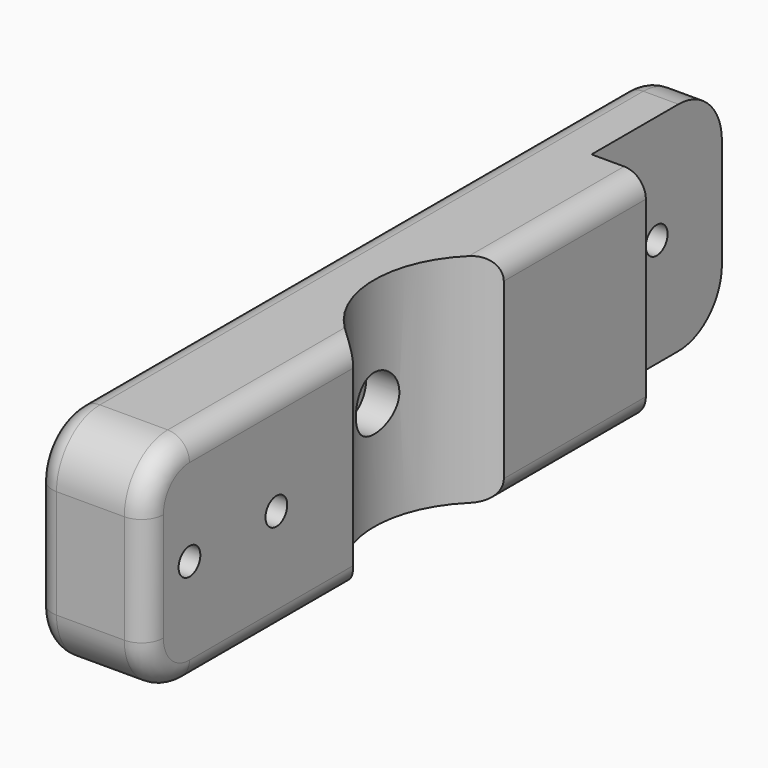
from build123d import *

# Parameters (mm, degrees)
F0_R     = 1.5875
F0_R_2   = 3.175
F1_DEPTH = 13
F2_W     = 6.35
F2_H     = 19.05
F3_DEPTH = 37.5
F4_R     = 6.35
F5_R     = 2.54
F6_SIZE  = 3.175


# Not quite as in the source:
# - a feature names something its author has since deleted; it is built from what else it names


with BuildPart() as f1:
    # F0 (on Right) → F1 (new body)
    with BuildSketch(Plane.YZ):
        Polygon((0, 0), (0, -12.7), (92.075, -12.7), (92.075, 0), (92.075, 12.7), (0, 12.7), align=None)
        with Locations((6.35, 0)):
            Circle(F0_R, mode=Mode.SUBTRACT)
        with Locations((19.05, 0)):
            Circle(F0_R, mode=Mode.SUBTRACT)
        with Locations((41.275, 0)):
            Circle(F0_R_2, mode=Mode.SUBTRACT)
        with Locations((82.55, 0)):
            Circle(F0_R, mode=Mode.SUBTRACT)
    extrude(amount=-F1_DEPTH)

    # F2 (on Top) → F3 (cut, symmetric)
    with BuildSketch(Plane.XY):
        with BuildLine():
            Line((0, 30.2764773719), (0, 52.2735226281))
            ThreePointArc((0, 52.2735226281), (-6.35, 41.275), (0, 30.2764773719))
        make_face()
        with Locations((-3.175, 82.55)):
            Rectangle(F2_W, F2_H)
    extrude(amount=F3_DEPTH, both=True, mode=Mode.SUBTRACT)

    # F4
    f4_edges = [f1.edges().sort_by_distance(p)[0] for p in [
        (-6.5, 0, -12.7),
        (-6.5, 0, 12.7),
        (-9.675, 92.075, -12.7),
        (-9.675, 92.075, 12.7),
    ]]
    fillet(f4_edges, radius=F4_R)

    # F5
    f5_edges = [f1.edges().sort_by_distance(p)[0] for p in [
        (-13, 90.215128, -10.840128),
        (-13, 92.075, 0),
        (0, 0, 0),
        (0, 62.649261, 12.7),
        (0, 62.649261, -12.7),
        (-13, 0, 0),
        (0, 1.859872, -10.840128),
        (0, 1.859872, 10.840128),
        (0, 18.313239, -12.7),
        (0, 18.313239, 12.7),
        (-13, 1.859872, -10.840128),
        (-13, 1.859872, 10.840128),
        (-13, 46.0375, -12.7),
        (-13, 90.215128, 10.840128),
        (-13, 46.0375, 12.7),
    ]]
    fillet(f5_edges, radius=F5_R)

    # F6
    f6_edges = [f1.edges().sort_by_distance(p)[0] for p in [
        (-13, 38.1, 0),
    ]]
    chamfer(f6_edges, length=F6_SIZE)


solid = f1.part
